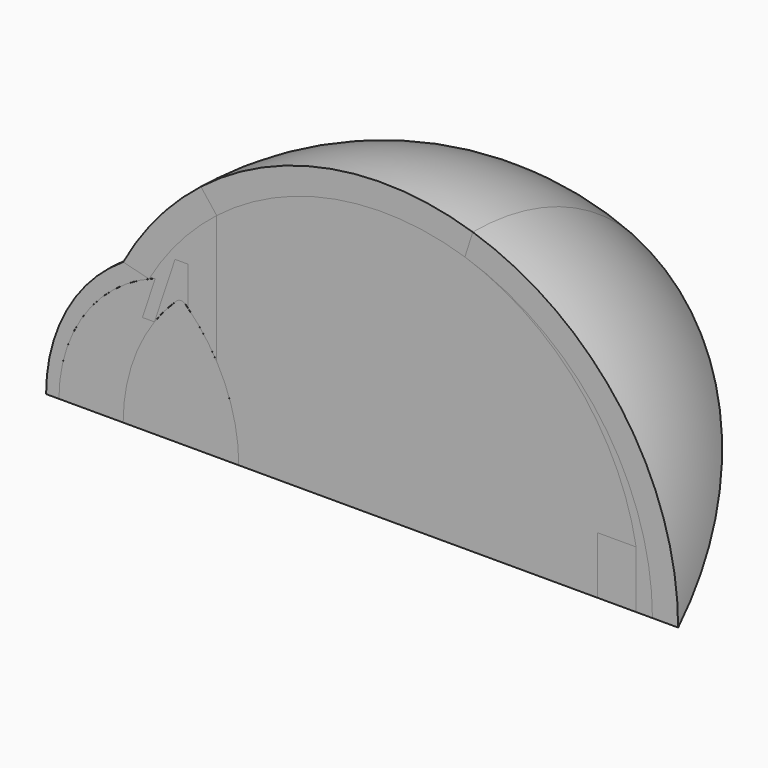
from build123d import *

# Parameters (mm, degrees)
F1_ANGLE  = 45
F3_ANGLE  = 45
F4_ANGLE  = 45
F6_ANGLE  = 45
F7_ANGLE  = 45
F9_ANGLE  = 45
F10_ANGLE = 45
F11_W     = 1.51221
F11_H     = 2.23
F12_ANGLE = 45
F13_ANGLE = 45
F15_ANGLE = 45
F16_ANGLE = 45
F19_ANGLE = 45
F22_ANGLE = 45
F25_ANGLE = 45
F28_ANGLE = 45
F31_ANGLE = 45


with BuildPart() as f1:
    # F0 (on Front) → F1 (revolve)
    with BuildSketch(Plane.XZ):
        with BuildLine():
            Line((-11.5, 0), (11.5, 0))
            ThreePointArc((11.5, 0), (2.8377537956, 11.1443776585), (-10.0995049384, 5.5))
            ThreePointArc((-10.0995049384, 5.5), (-12.3007384778, 3.1324910215), (-13.0995049384, 0))
            Line((-13.0995049384, 0), (-11.5, 0))
        make_face()
    revolve(axis=Axis((0, 0, 0), (-1, 0, 0)), revolution_arc=F1_ANGLE)

    # F2 (on Front) → F3 (revolve, cut)
    with BuildSketch(Plane.XZ):
        with BuildLine():
            ThreePointArc((11.5, 0), (2.8377537956, 11.1443776585), (-10.0995049384, 5.5))
            Line((-10.0995049384, 5.5), (-9.0932667397, 5.25))
            ThreePointArc((-9.0932667397, 5.25), (2.7175999736, 10.142221176), (10.5, 0))
            Line((10.5, 0), (11.5, 0))
        make_face()
    revolve(axis=Axis((0, 0, 0), (-1, 0, 0)), revolution_arc=F3_ANGLE, mode=Mode.SUBTRACT)

    # F5 (on face) → F6 (revolve, cut)
    with BuildSketch(Plane.XZ):
        with BuildLine():
            ThreePointArc((-12.5995049384, 0), (-11.6423500551, 3.1565885979), (-9.0932667397, 5.25))
            Line((-9.0932667397, 5.25), (-10.0995049384, 5.5))
            ThreePointArc((-10.0995049384, 5.5), (-12.3007384778, 3.1324910215), (-13.0995049384, 0))
            Line((-13.0995049384, 0), (-12.5995049384, 0))
        make_face()
    revolve(axis=Axis((-12.2997524692, 0, 0), (-1, 0, 0)), revolution_arc=F6_ANGLE, mode=Mode.SUBTRACT)

    # F8 (on Front) → F9 (revolve, cut)
    with BuildSketch(Plane.XZ):
        with BuildLine():
            ThreePointArc((3.2015621187, 10), (8.2807192075, 6.1420955145), (10, 0))
            Line((10, 0), (10.5, 0))
            ThreePointArc((10.5, 0), (8.4813442993, 6.1900564518), (3.2015621187, 10))
        make_face()
    revolve(axis=Axis((0, 0, 0), (-1, 0, 0)), revolution_arc=F9_ANGLE, mode=Mode.SUBTRACT)

    # F11 (on face) → F12 (revolve, cut)
    with BuildSketch(Plane.XZ):
        with Locations((9.1086225685, 1.115)):
            Rectangle(F11_W, F11_H)
    revolve(axis=Axis((9.1086225685, 0, 0), (-1, 0, 0)), revolution_arc=F12_ANGLE, mode=Mode.SUBTRACT)

    # F14 (on Front) → F15 (revolve, cut)
    with BuildSketch(Plane.XZ):
        with BuildLine():
            ThreePointArc((10, 0), (9.9947523902, 1.1187845105), (9.8647275685, 2.23))
            Line((9.8647275685, 2.23), (9.8647275685, 0))
            Line((9.8647275685, 0), (10, 0))
        make_face()
    revolve(axis=Axis((9.9323637842, 0, 0), (-1, 0, 0)), revolution_arc=F15_ANGLE, mode=Mode.SUBTRACT)

    # F20 (on Front) → F21 (revolve, cut)
    with BuildSketch(Plane.XZ):
        with BuildLine():
            Line((-9.3495049384, 3.8445862413), (-8.8495049384, 5.3445862413))
            ThreePointArc((-8.8495049384, 5.3445862413), (-11.5684914777, 3.2644717065), (-12.5995049384, 0))
            Line((-12.5995049384, 0), (-8.8495049384, 0))
            Line((-8.8495049384, 0), (-8.8495049384, 3.8445862413))
            Line((-8.8495049384, 3.8445862413), (-9.3495049384, 3.8445862413))
        make_face()
    revolve(axis=Axis((-10.7245049384, 0, 0), (1, 0, 0)), mode=Mode.SUBTRACT)


with BuildPart() as f4:
    # F2 (on Front) → F4 (revolve)
    with BuildSketch(Plane.XZ):
        with BuildLine():
            ThreePointArc((11.5, 0), (2.8377537956, 11.1443776585), (-10.0995049384, 5.5))
            Line((-10.0995049384, 5.5), (-9.0932667397, 5.25))
            ThreePointArc((-9.0932667397, 5.25), (2.7175999736, 10.142221176), (10.5, 0))
            Line((10.5, 0), (11.5, 0))
        make_face()
    revolve(axis=Axis((0, 0, 0), (-1, 0, 0)), revolution_arc=F4_ANGLE)

    # F17 (on Front) → F18 (revolve, cut)
    with BuildSketch(Plane.XZ):
        with BuildLine():
            ThreePointArc((11.5, 0), (9.2890913754, 6.7795856377), (3.5064727967, 10.9523809524))
            Line((3.5064727967, 10.9523809524), (3.2015621187, 10))
            ThreePointArc((3.2015621187, 10), (8.4813442993, 6.1900564518), (10.5, 0))
            Line((10.5, 0), (11.5, 0))
        make_face()
    revolve(axis=Axis((11, 0, 0), (1, 0, 0)), mode=Mode.SUBTRACT)

    # F29 (on Front) → F30 (revolve, cut)
    with BuildSketch(Plane.XZ):
        with BuildLine():
            ThreePointArc((-9.0932667397, 5.25), (-7.9222484154, 6.8911523017), (-6.4591549508, 8.2782436134))
            Line((-6.4591549508, 8.2782436134), (-7.0743125651, 9.066647767))
            ThreePointArc((-7.0743125651, 9.066647767), (-8.7701337495, 7.438733361), (-10.0995049384, 5.5))
            Line((-10.0995049384, 5.5), (-9.0932667397, 5.25))
        make_face()
    revolve(axis=Axis((-7.8495049384, 0, 0), (-1, 0, 0)), mode=Mode.SUBTRACT)


with BuildPart() as f7:
    # F5 (on face) → F7 (revolve)
    with BuildSketch(Plane.XZ):
        with BuildLine():
            ThreePointArc((-12.5995049384, 0), (-11.6423500551, 3.1565885979), (-9.0932667397, 5.25))
            Line((-9.0932667397, 5.25), (-10.0995049384, 5.5))
            ThreePointArc((-10.0995049384, 5.5), (-12.3007384778, 3.1324910215), (-13.0995049384, 0))
            Line((-13.0995049384, 0), (-12.5995049384, 0))
        make_face()
    revolve(axis=Axis((0, 0, 0), (-1, 0, 0)), revolution_arc=F7_ANGLE)


with BuildPart() as f10:
    # F8 (on Front) → F10 (revolve)
    with BuildSketch(Plane.XZ):
        with BuildLine():
            ThreePointArc((3.2015621187, 10), (8.2807192075, 6.1420955145), (10, 0))
            Line((10, 0), (10.5, 0))
            ThreePointArc((10.5, 0), (8.4813442993, 6.1900564518), (3.2015621187, 10))
        make_face()
    revolve(axis=Axis((10.25, 0, 0), (-1, 0, 0)), revolution_arc=F10_ANGLE)

    # F14 (on Front) → F16 (revolve)
    with BuildSketch(Plane.XZ):
        with BuildLine():
            ThreePointArc((10, 0), (9.9947523902, 1.1187845105), (9.8647275685, 2.23))
            Line((9.8647275685, 2.23), (9.8647275685, 0))
            Line((9.8647275685, 0), (10, 0))
        make_face()
    revolve(axis=Axis((0, 0, 0), (-1, 0, 0)), revolution_arc=F16_ANGLE)


with BuildPart() as f13:
    # F11 (on face) → F13 (revolve)
    with BuildSketch(Plane.XZ):
        with Locations((9.1086225685, 1.115)):
            Rectangle(F11_W, F11_H)
    revolve(axis=Axis((0, 0, 0), (-1, 0, 0)), revolution_arc=F13_ANGLE)


with BuildPart() as f19:
    # F17 (on Front) → F19 (revolve)
    with BuildSketch(Plane.XZ):
        with BuildLine():
            ThreePointArc((11.5, 0), (9.2890913754, 6.7795856377), (3.5064727967, 10.9523809524))
            Line((3.5064727967, 10.9523809524), (3.2015621187, 10))
            ThreePointArc((3.2015621187, 10), (8.4813442993, 6.1900564518), (10.5, 0))
            Line((10.5, 0), (11.5, 0))
        make_face()
    revolve(axis=Axis((0, 0, 0), (-1, 0, 0)), revolution_arc=F19_ANGLE)


with BuildPart() as f22:
    # F20 (on Front) → F22 (revolve)
    with BuildSketch(Plane.XZ):
        with BuildLine():
            Line((-9.3495049384, 3.8445862413), (-8.8495049384, 5.3445862413))
            ThreePointArc((-8.8495049384, 5.3445862413), (-11.5684914777, 3.2644717065), (-12.5995049384, 0))
            Line((-12.5995049384, 0), (-8.8495049384, 0))
            Line((-8.8495049384, 0), (-8.8495049384, 3.8445862413))
            Line((-8.8495049384, 3.8445862413), (-9.3495049384, 3.8445862413))
        make_face()
    revolve(axis=Axis((0, 0, 0), (-1, 0, 0)), revolution_arc=F22_ANGLE)


with BuildPart() as f24_tool:
    # F23 (on Front) → F24 (revolve)
    with BuildSketch(Plane.XZ):
        with BuildLine():
            Line((-10.0995049384, 0), (-5.5995049384, 0))
            ThreePointArc((-5.5995049384, 0), (-6.1408791354, 2.6344401261), (-7.6772587181, 4.8419044128))
            ThreePointArc((-7.6772587181, 4.8419044128), (-7.8495049384, 4.9107104847), (-8.0217511587, 4.8419044128))
            ThreePointArc((-8.0217511587, 4.8419044128), (-9.5581307413, 2.6344401261), (-10.0995049384, 0))
        make_face()
    revolve(axis=Axis((0, 0, 0), (-1, 0, 0)))


with BuildPart() as f1_1:
    add(f1.part)

    # F24: cut by f24_tool
    add(f24_tool.part, mode=Mode.SUBTRACT)

    # F26 (on Front) → F27 (revolve, cut)
    with BuildSketch(Plane.XZ):
        with BuildLine():
            Line((-8.8495049384, 5.3445862413), (-9.3495049384, 3.8445862413))
            Line((-9.3495049384, 3.8445862413), (-8.8823713109, 3.8445862413))
            Line((-8.8823713109, 3.8445862413), (-8.0810395972, 6.2485813822))
            Line((-8.0810395972, 6.2485813822), (-7.5810395972, 6.2485813822))
            Line((-7.5810395972, 6.2485813822), (-7.5810395972, 4.7485813822))
            ThreePointArc((-7.5810395972, 4.7485813822), (-6.9689696113, 4.0524234931), (-6.4591549508, 3.2782436134))
            Line((-6.4591549508, 3.2782436134), (-6.4591549508, 8.2782436134))
            ThreePointArc((-6.4591549508, 8.2782436134), (-7.9222484154, 6.8911523017), (-9.0932667397, 5.25))
            ThreePointArc((-9.0932667397, 5.25), (-8.9719298306, 5.298695062), (-8.8495049384, 5.3445862413))
        make_face()
    revolve(axis=Axis((-7.8495049384, 0, 0), (-1, 0, 0)), mode=Mode.SUBTRACT)


with BuildPart() as f22_1:
    add(f22.part)

    # F24: cut by f24_tool
    add(f24_tool.part, mode=Mode.SUBTRACT)


with BuildPart() as f25:
    # F23 (on Front) → F25 (revolve)
    with BuildSketch(Plane.XZ):
        with BuildLine():
            Line((-10.0995049384, 0), (-5.5995049384, 0))
            ThreePointArc((-5.5995049384, 0), (-6.1408791354, 2.6344401261), (-7.6772587181, 4.8419044128))
            ThreePointArc((-7.6772587181, 4.8419044128), (-7.8495049384, 4.9107104847), (-8.0217511587, 4.8419044128))
            ThreePointArc((-8.0217511587, 4.8419044128), (-9.5581307413, 2.6344401261), (-10.0995049384, 0))
        make_face()
    revolve(axis=Axis((0, 0, 0), (-1, 0, 0)), revolution_arc=F25_ANGLE)


with BuildPart() as f28:
    # F26 (on Front) → F28 (revolve)
    with BuildSketch(Plane.XZ):
        with BuildLine():
            Line((-8.8495049384, 5.3445862413), (-9.3495049384, 3.8445862413))
            Line((-9.3495049384, 3.8445862413), (-8.8823713109, 3.8445862413))
            Line((-8.8823713109, 3.8445862413), (-8.0810395972, 6.2485813822))
            Line((-8.0810395972, 6.2485813822), (-7.5810395972, 6.2485813822))
            Line((-7.5810395972, 6.2485813822), (-7.5810395972, 4.7485813822))
            ThreePointArc((-7.5810395972, 4.7485813822), (-6.9689696113, 4.0524234931), (-6.4591549508, 3.2782436134))
            Line((-6.4591549508, 3.2782436134), (-6.4591549508, 8.2782436134))
            ThreePointArc((-6.4591549508, 8.2782436134), (-7.9222484154, 6.8911523017), (-9.0932667397, 5.25))
            ThreePointArc((-9.0932667397, 5.25), (-8.9719298306, 5.298695062), (-8.8495049384, 5.3445862413))
        make_face()
    revolve(axis=Axis((-7.8495049384, 0, 0), (-1, 0, 0)), revolution_arc=F28_ANGLE)


with BuildPart() as f31:
    # F29 (on Front) → F31 (revolve)
    with BuildSketch(Plane.XZ):
        with BuildLine():
            ThreePointArc((-9.0932667397, 5.25), (-7.9222484154, 6.8911523017), (-6.4591549508, 8.2782436134))
            Line((-6.4591549508, 8.2782436134), (-7.0743125651, 9.066647767))
            ThreePointArc((-7.0743125651, 9.066647767), (-8.7701337495, 7.438733361), (-10.0995049384, 5.5))
            Line((-10.0995049384, 5.5), (-9.0932667397, 5.25))
        make_face()
    revolve(axis=Axis((-7.8495049384, 0, 0), (-1, 0, 0)), revolution_arc=F31_ANGLE)


solid = Compound([f4.part, f7.part, f10.part, f13.part, f19.part, f1_1.part, f22_1.part, f25.part, f28.part, f31.part])
